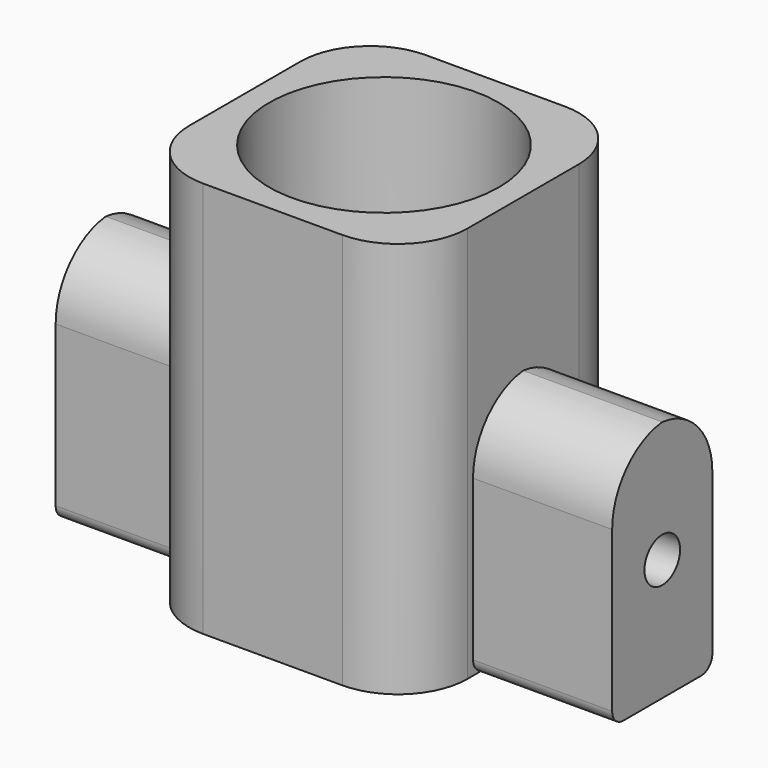
from build123d import *

# Parameters (mm, degrees)
F0_W         = 20
F0_H         = 20
F0_R         = 8.25
F1_DEPTH     = 28.5
F0_R_2       = 4.75
F2_DEPTH     = 1.5
F3_W         = 9
F3_H         = 17.5
F3_R         = 1.6
F4_DEPTH     = 10
F5_W         = 9
F5_H         = 17.5
F6_DEPTH     = 10
F7_DEPTH     = 30.001
F8_R         = 5
F9_T1_DEPTH  = 22.5
F10_T1_DEPTH = 22.5
F11_R        = 1


# Not quite as in the source:
# - a fillet or chamfer that OpenCascade refuses, or shapes differently, is made with other operations: its cross-section is extruded or revolved along the edge and cut away or added


with BuildPart() as f1:
    # F0 (on Top) → F1 (new body)
    with BuildSketch(Plane.XY):
        Rectangle(F0_W, F0_H)
        Circle(F0_R, mode=Mode.SUBTRACT)
    extrude(amount=F1_DEPTH)

    # F0 (on Top) → F2 (join)
    with BuildSketch(Plane.XY):
        Circle(F0_R)
        Circle(F0_R_2, mode=Mode.SUBTRACT)
    extrude(amount=F2_DEPTH)

    # F3 (on face) → F4 (join)
    with BuildSketch(Plane(origin=(-10, 0, 0), x_dir=(0, -1, 0), z_dir=(-1, 0, 0))):
        with Locations((0, 8.75)):
            Rectangle(F3_W, F3_H)
        with Locations((0, 8.75)):
            Circle(F3_R, mode=Mode.SUBTRACT)
    extrude(amount=F4_DEPTH)

    # F5 (on face) → F6 (join)
    with BuildSketch(Plane.YZ.offset(10)):
        with Locations((0, 8.75)):
            Rectangle(F5_W, F5_H)
    extrude(amount=F6_DEPTH)

    # F3 (on face) → F7 (cut, through all)
    with BuildSketch(Plane(origin=(-10, 0, 0), x_dir=(0, -1, 0), z_dir=(-1, 0, 0))):
        with Locations((0, 8.75)):
            Circle(F3_R)
    extrude(amount=-F7_DEPTH, mode=Mode.SUBTRACT)

    # F8
    f8_edges = [f1.edges().sort_by_distance(p)[0] for p in [
        (-10, -10, 14.25),
        (10, -10, 14.25),
        (10, 10, 14.25),
        (-10, 10, 14.25),
    ]]
    fillet(f8_edges, radius=F8_R)

    # F9: fillet of radius 5 on 2 edges, made by hand

    # F9_s2 → F9_t1 (cut)
    with BuildSketch(Plane.YZ.offset(10)):
        with BuildLine():
            ThreePointArc((-4.5, 12.5), (-3.0355339059, 16.0355339059), (0.5, 17.5))
            Line((0.5, 17.5), (-4.5, 17.5))
            Line((-4.5, 17.5), (-4.5, 12.5))
        make_face()
        with BuildLine():
            ThreePointArc((-0.5, 17.5), (3.0355339059, 16.0355339059), (4.5, 12.5))
            Line((4.5, 12.5), (4.5, 17.5))
            Line((4.5, 17.5), (-0.5, 17.5))
        make_face()
    extrude(amount=F9_T1_DEPTH, mode=Mode.SUBTRACT)

    # F10: fillet of radius 5 on 2 edges, made by hand

    # F10_s2 → F10_t1 (cut)
    with BuildSketch(Plane.YZ.offset(-32.5)):
        with BuildLine():
            ThreePointArc((-4.5, 12.5), (-3.0355339059, 16.0355339059), (0.5, 17.5))
            Line((0.5, 17.5), (-4.5, 17.5))
            Line((-4.5, 17.5), (-4.5, 12.5))
        make_face()
        with BuildLine():
            ThreePointArc((4.5, 12.5), (3.0355339059, 16.0355339059), (-0.5, 17.5))
            Line((-0.5, 17.5), (4.5, 17.5))
            Line((4.5, 17.5), (4.5, 12.5))
        make_face()
    extrude(amount=F10_T1_DEPTH, mode=Mode.SUBTRACT)

    # F11
    f11_edges = [f1.edges().sort_by_distance(p)[0] for p in [
        (15, -4.5, 0),
        (15, 4.5, 0),
        (-15, 4.5, 0),
        (-15, -4.5, 0),
    ]]
    fillet(f11_edges, radius=F11_R)


solid = f1.part
